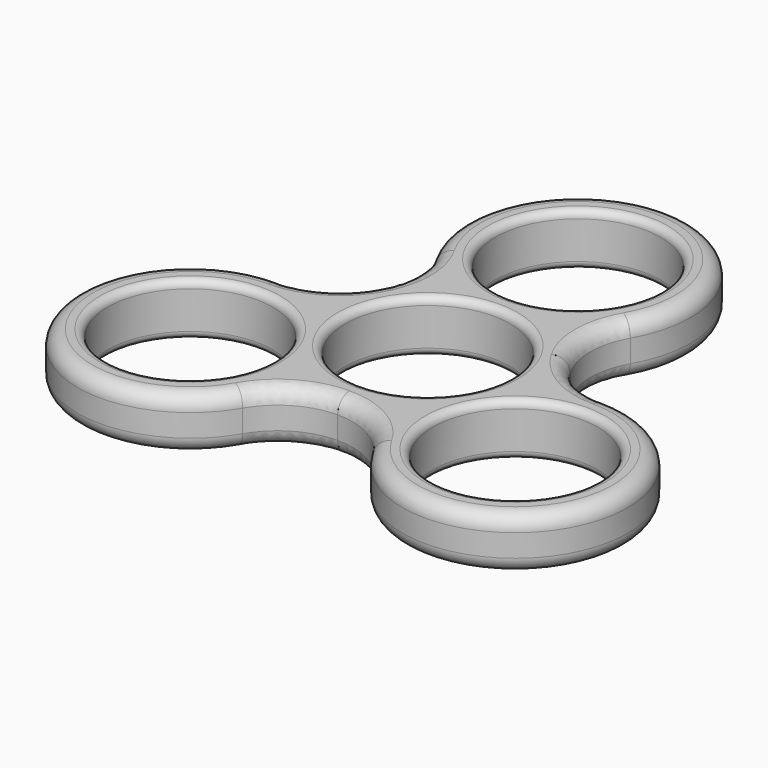
from build123d import *

# Parameters (mm, degrees)
F0_R     = 11
F1_DEPTH = 7
F2_R     = 9.999
F3_R     = 2
F4_R     = 1


# Not quite as in the source:
# - a fillet or chamfer is up to 0.001 mm smaller than in the source, because OpenCascade refuses the exact size


with BuildPart() as f1:
    # F0 (on Top) → F1 (new body)
    with BuildSketch(Plane.XY):
        with BuildLine():
            ThreePointArc((8.2915619759, 12.5), (0, 40), (-8.2915619759, 12.5))
            ThreePointArc((-8.2915619759, 12.5), (-12.9903810568, 7.5), (-14.9710985352, 0.9307033082))
            ThreePointArc((-14.9710985352, 0.9307033082), (-34.6410161514, -20), (-6.6795365594, -13.4307033082))
            ThreePointArc((-6.6795365594, -13.4307033082), (0, -15), (6.6795365594, -13.4307033082))
            ThreePointArc((6.6795365594, -13.4307033082), (34.6410161514, -20), (14.9710985352, 0.9307033082))
            ThreePointArc((14.9710985352, 0.9307033082), (12.9903810568, 7.5), (8.2915619759, 12.5))
        make_face()
        with Locations((-21.6506350946, -12.5)):
            Circle(F0_R, mode=Mode.SUBTRACT)
        Circle(F0_R, mode=Mode.SUBTRACT)
        with Locations((21.6506350946, -12.5)):
            Circle(F0_R, mode=Mode.SUBTRACT)
        with Locations((0, 25)):
            Circle(F0_R, mode=Mode.SUBTRACT)
    extrude(amount=F1_DEPTH)

    # F2 (radius 10 in the source; OpenCascade refuses exactly that, so slightly less here)
    f2_edges = [f1.edges().sort_by_distance(p)[0] for p in [
        (8.291562, 12.5, 3.5),
        (14.971099, 0.930703, 3.5),
        (-6.679537, -13.430703, 3.5),
        (6.679537, -13.430703, 3.5),
        (-8.291562, 12.5, 3.5),
        (-14.971099, 0.930703, 3.5),
    ]]
    fillet(f2_edges, radius=F2_R)

    # F3
    f3_edges = [f1.edges().sort_by_distance(p)[0] for p in [
        (-34.641016, -20, 0),
        (-11.65048, 12.5, 7),
    ]]
    fillet(f3_edges, radius=F3_R)

    # F4
    f4_edges = [f1.edges().sort_by_distance(p)[0] for p in [
        (10.650635, -12.5, 7),
        (-11, 0, 7),
        (-32.650635, -12.5, 7),
        (-11, 25, 7),
        (-32.650635, -12.5, 0),
        (10.650635, -12.5, 0),
        (-11, 0, 0),
        (-11, 25, 0),
    ]]
    fillet(f4_edges, radius=F4_R)


solid = f1.part
